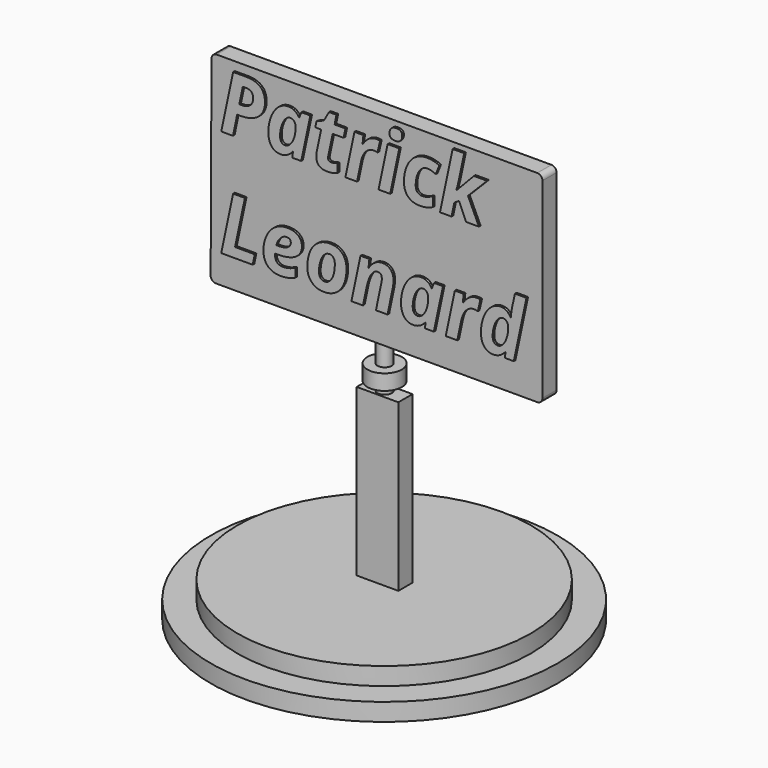
from build123d import *

# Parameters (mm, degrees)
F1_DEPTH     = 43.3216542006
F0_W         = 101.8618196249
F0_H         = 406.3027203083
F2_TEXT_SIZE = 192.7126405968
F3_DEPTH     = 5.08
F5_DEPTH     = 14.478
F6_R         = 358.8673810864
F6_W         = 101.8618196249
F6_H         = 43.3216542006
F7_DEPTH     = 43.18
F8_R         = 424.2013179967
F8_R_2       = 358.8673810864
F9_DEPTH     = 43.18
F10_R        = 12.7
F11_R        = 17.599135576
F12_DEPTH    = 17.272
F13_R        = 17.2514261767
F14_DEPTH    = 57.15
F15_R        = 42.0684917016
F15_R_2      = 17.2514261767
F16_DEPTH    = 18.8975296915
F17_R        = 17.2978744673
F18_DEPTH    = 111.76
F19_R        = 19.812
F20_DEPTH    = 41.91


# Not quite as in the source:
# - Text() gives the source's letters only with a copy of the font that has no kerning and outlines rounded to 1/6400 em; it was checked with that copy


with BuildPart() as f1:
    # F0 (on Front) → F1 (new body)
    with BuildSketch(Plane.XZ):
        Polygon((-178.3141490915, 158.7198749185), (-180.51828444, -334.9961638451), (631.4799189568, -334.9961638451), (631.4799189568, 158.7198749185), align=None)
    extrude(amount=-F1_DEPTH)

    # F2 (on face) → F3 (join)
    with BuildSketch(Plane.XZ):
        with Locations((-155.4256379604, 0)):
            Text('Patrick', F2_TEXT_SIZE, font='Open Sans', font_style=FontStyle.BOLDITALIC, text_align=(TextAlign.LEFT, TextAlign.BOTTOM))
        with Locations((-155.4256379604, -262.0891912116)):
            Text('Leonard', F2_TEXT_SIZE, font='Open Sans', font_style=FontStyle.BOLDITALIC, text_align=(TextAlign.LEFT, TextAlign.BOTTOM))
    extrude(amount=F3_DEPTH)

    # F4 (on face) → F5 (join)
    with BuildSketch(Plane(origin=(0, 43.3216542006, 0), x_dir=(-1, 0, 0), z_dir=(0, 1, 0))):
        with BuildLine():
            ThreePointArc((-471.9009101391, 78.4758478403), (-491.323751898, -26.0441303253), (-471.9009101391, -130.5641084909))
            ThreePointArc((-471.9009101391, -130.5641084909), (-392.3729362457, -252.6742309068), (-254.478007555, -299.7971475124))
            ThreePointArc((-254.478007555, -299.7971475124), (-119.2006052928, -248.9883283341), (-36.3922975957, -130.5641084909))
            ThreePointArc((-36.3922975957, -130.5641084909), (-19.3951484189, -24.6916024136), (-48.6247195985, 78.4758478403))
            ThreePointArc((-48.6247195985, 78.4758478403), (-58.4237814551, 91.4402649122), (-72.4166482687, 99.7044891119))
            ThreePointArc((-72.4166482687, 99.7044891119), (-95.2314134987, -36.431227076), (-198.5018700361, -128.0208528042))
            ThreePointArc((-198.5018700361, -128.0208528042), (-218.5277246318, -65.4766158256), (-223.5902547836, 0))
            ThreePointArc((-223.5902547836, 0), (-207.4346558282, 28.4618424712), (-177.2732287645, 41.164919734))
            Line((-177.2732287645, 41.164919734), (-204.9347907305, 63.9245905664))
            ThreePointArc((-204.9347907305, 63.9245905664), (-229.3126291538, 58.6514513614), (-250.6085038185, 45.6679724157))
            Line((-250.6085038185, 45.6679724157), (-230.023175478, 86.8386551738))
            Line((-230.023175478, 86.8386551738), (-262.8310620785, 124.1495758295))
            Line((-262.8310620785, 124.1495758295), (-296.2822318077, 86.8386551738))
            Line((-296.2822318077, 86.8386551738), (-282.7731072903, 45.6679724157))
            ThreePointArc((-282.7731072903, 45.6679724157), (-302.4935809573, 58.3036134607), (-325.2303600311, 63.9245905664))
            Line((-325.2303600311, 63.9245905664), (-363.1846010685, 41.164919734))
            ThreePointArc((-363.1846010685, 41.164919734), (-330.4524692677, 30.6721761364), (-314.937710762, 0))
            ThreePointArc((-314.937710762, 0), (-316.3991139197, -64.5689756058), (-328.4468352795, -128.0208528042))
            ThreePointArc((-328.4468352795, -128.0208528042), (-427.8632071256, -34.8119578164), (-449.6998415203, 99.7044891119))
            ThreePointArc((-449.6998415203, 99.7044891119), (-462.1740553611, 90.5267725973), (-471.9009101391, 78.4758478403))
        make_face()
    extrude(amount=F5_DEPTH)

    # F10
    f10_edges = [f1.edges().sort_by_distance(p)[0] for p in [
        (631.479919, 21.660827, 158.719875),
        (631.479919, 21.660827, -334.996164),
        (-180.518284, 21.660827, -334.996164),
        (-178.314149, 21.660827, 158.719875),
    ]]
    fillet(f10_edges, radius=F10_R)

    # F19 (on face) → F20 (cut)
    with BuildSketch(Plane(origin=(0, 0, -334.9961638451), x_dir=(1, 0, 0), z_dir=(0, 0, -1))):
        with Locations((230.1296591759, -21.6608271003)):
            Circle(F19_R)
    extrude(amount=-F20_DEPTH, mode=Mode.SUBTRACT)


with BuildPart() as f1b:
    # F0 (on Front) → F1, piece 2 (new body)
    with BuildSketch(Plane.XZ):
        with Locations((227.9675081372, -648.9985436201)):
            Rectangle(F0_W, F0_H)
    extrude(amount=-F1_DEPTH)

    # F6 (on face) → F7 (join)
    with BuildSketch(Plane(origin=(0, 0, -852.1499037743), x_dir=(1, 0, 0), z_dir=(0, 0, -1))):
        with Locations((227.9675081372, -20.1313402504)):
            Circle(F6_R)
        with Locations((227.9675081372, -21.6608271003)):
            Rectangle(F6_W, F6_H, mode=Mode.SUBTRACT)
        with Locations((227.9675081372, -21.6608271003)):
            Rectangle(F6_W, F6_H)
    extrude(amount=F7_DEPTH)

    # F8 (on face) → F9 (join)
    with BuildSketch(Plane(origin=(0, 0, -895.3299037743), x_dir=(1, 0, 0), z_dir=(0, 0, -1))):
        with Locations((227.9675081372, -20.1313402504)):
            Circle(F8_R)
        with Locations((227.9675081372, -20.1313402504)):
            Circle(F8_R_2, mode=Mode.SUBTRACT)
        with Locations((227.9675081372, -20.1313402504)):
            Circle(F8_R_2)
    extrude(amount=F9_DEPTH)

    # F11 (on face) → F12 (cut)
    with BuildSketch(Plane.XY.offset(-445.847183466)):
        with Locations((227.9675081372, 21.6608271003)):
            Circle(F11_R)
    extrude(amount=-F12_DEPTH, mode=Mode.SUBTRACT)

    # F13 (on face) → F14 (join)
    with BuildSketch(Plane.XY.offset(-463.119183466)):
        with Locations((227.9675081372, 21.6608271003)):
            Circle(F13_R)
    extrude(amount=F14_DEPTH)

    # F15 (on face) → F16 (join, symmetric)
    with BuildSketch(Plane.XY.offset(-405.969183466)):
        with Locations((227.9675081372, 21.6608271003)):
            Circle(F15_R)
        with Locations((227.9675081372, 21.6608271003)):
            Circle(F15_R_2, mode=Mode.SUBTRACT)
    extrude(amount=F16_DEPTH, both=True)

    # F17 (on face) → F18 (join)
    with BuildSketch(Plane.XY.offset(-405.969183466)):
        with Locations((227.9675081372, 21.6608271003)):
            Circle(F17_R)
    extrude(amount=F18_DEPTH)


solid = Compound([f1.part, f1b.part])
